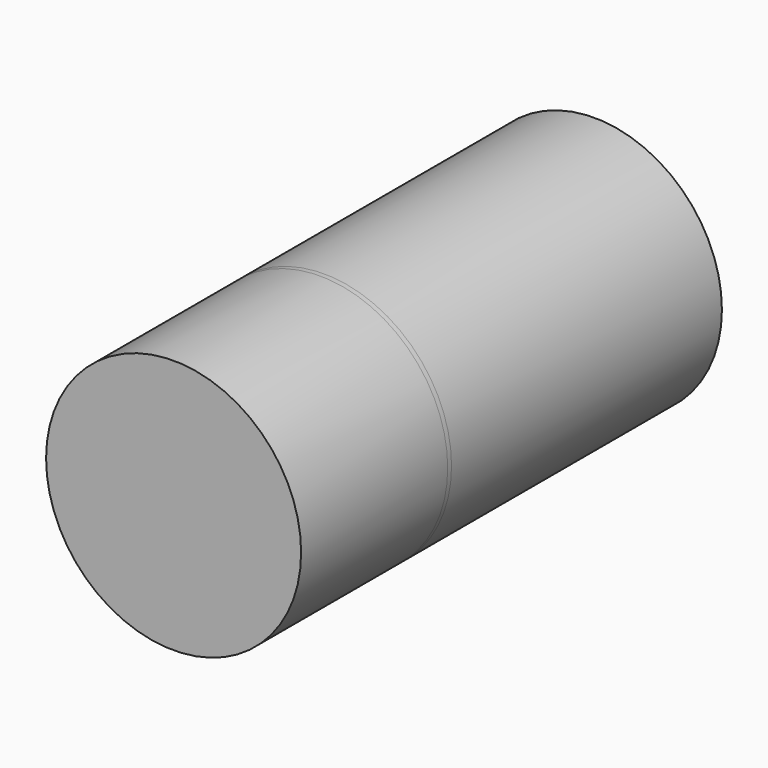
from build123d import *

# Parameters (mm, degrees)
F1_R     = 13.608601514
F2_DEPTH = 36.068
F4_DEPTH = 36.576
F5_DEPTH = 56.134


# Not quite as in the source:
# - the program builds the solid bodies; features that only make, move or delete a surface that nothing else refers to are left out


with BuildPart() as f2:
    # F1 (on Front) → F2 (new body)
    with BuildSketch(Plane.XZ):
        Circle(F1_R)
    extrude(amount=-F2_DEPTH)

    # F4 (add): a face of the model
    f4_faces = [f2.faces().sort_by_distance(p)[0] for p in [
        (0, 36.068, 0),
    ]]
    extrude(f4_faces, amount=-F4_DEPTH)

    # F5 (add): a face of the model
    f5_faces = [f2.faces().sort_by_distance(p)[0] for p in [
        (0, 36.068, 0),
    ]]
    extrude(f5_faces, amount=-F5_DEPTH)


solid = f2.part
